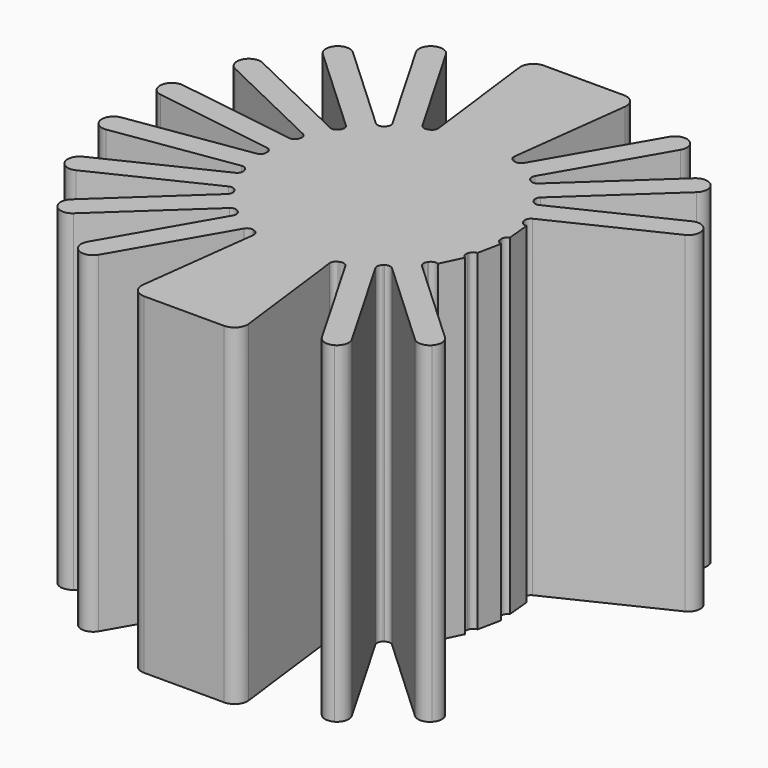
from build123d import *

# Parameters (mm, degrees)
F1_DEPTH = 14
F2_R     = 0.49999
F3_R     = 0.25
F4_R     = 0.55
F6_DEPTH = 14.001


# Not quite as in the source:
# - a fillet or chamfer is up to 0.001 mm smaller than in the source, because OpenCascade refuses the exact size
# - ends of sketch curves that miss each other by under 0.0002 mm in the source are joined


with BuildPart() as f1:
    # F0 (on Top) → F1 (new body)
    with BuildSketch(Plane.XY):
        with BuildLine():
            ThreePointArc((4.9441205719, -0.2411882471), (4.9485299247, -0.1206299488), (4.95, 0))
            ThreePointArc((4.95, 0), (4.9485691313, 0.1190107267), (4.9442773523, 0.2379526499))
            ThreePointArc((4.9442773523, 0.2379526499), (4.894953731, 0.7361575721), (4.7955586509, 1.2268321915))
            ThreePointArc((4.7955586509, 1.2268321915), (4.7305625494, 1.4574902971), (4.6544792073, 1.6847324146))
            ThreePointArc((4.6544792073, 1.6847324146), (4.4604984174, 2.1462650974), (4.2208902988, 2.585843206))
            ThreePointArc((4.2208902988, 2.585843206), (4.0907941216, 2.7870958819), (3.9511101589, 2.9818163109))
            ThreePointArc((3.9511101589, 2.9818163109), (3.6297082448, 3.36566755), (3.2711773205, 3.7150907038))
            ThreePointArc((3.2711773205, 3.7150907038), (3.0875406838, 3.8690557667), (2.8966676337, 4.0139527426))
            ThreePointArc((2.8966676337, 4.0139527426), (2.476402566, 4.2860156709), (2.030805882, 4.5142360893))
            ThreePointArc((2.030805882, 4.5142360893), (1.8088052095, 4.6076809475), (1.5825217056, 4.6902158854))
            ThreePointArc((1.5825217056, 4.6902158854), (0, 4.95), (-1.5825217056, 4.6902158854))
            ThreePointArc((-1.5825217056, 4.6902158854), (-1.8088052095, 4.6076809475), (-2.030805882, 4.5142360893))
            ThreePointArc((-2.030805882, 4.5142360893), (-2.476402566, 4.2860156709), (-2.8966676337, 4.0139527426))
            ThreePointArc((-2.8966676337, 4.0139527426), (-3.0875406838, 3.8690557667), (-3.2711773205, 3.7150907038))
            ThreePointArc((-3.2711773205, 3.7150907038), (-3.6297082448, 3.36566755), (-3.9511101589, 2.9818163109))
            ThreePointArc((-3.9511101589, 2.9818163109), (-4.0907941216, 2.7870958819), (-4.2208902988, 2.585843206))
            ThreePointArc((-4.2208902988, 2.585843206), (-4.4604984174, 2.1462650974), (-4.6544792073, 1.6847324146))
            ThreePointArc((-4.6544792073, 1.6847324146), (-4.7305625494, 1.4574902971), (-4.7955586509, 1.2268321915))
            ThreePointArc((-4.7955586509, 1.2268321915), (-4.894953731, 0.7361575721), (-4.9442773523, 0.2379526499))
            ThreePointArc((-4.9442773523, 0.2379526499), (-4.949999735, -0.0016196967), (-4.9441205719, -0.2411882471))
            ThreePointArc((-4.9441205719, -0.2411882471), (-4.8944709245, -0.7393607841), (-4.7947547569, -1.229970252))
            ThreePointArc((-4.7947547569, -1.229970252), (-4.7296077214, -1.4605857733), (-4.6533756832, -1.6877780515))
            ThreePointArc((-4.6533756832, -1.6877780515), (-4.4590928973, -2.14918369), (-4.21919716, -2.5886048994))
            ThreePointArc((-4.21919716, -2.5886048994), (-4.0889693063, -2.7897723944), (-3.949157944, -2.9844013693))
            ThreePointArc((-3.949157944, -2.9844013693), (-3.6275048978, -3.3680421934), (-3.2687453797, -3.7172306416))
            ThreePointArc((-3.2687453797, -3.7172306416), (-3.0850080241, -3.8710754954), (-2.894040191, -4.0158475286))
            ThreePointArc((-2.894040191, -4.0158475286), (-2.473597169, -4.2876353676), (-2.0278512278, -4.5155641284))
            ThreePointArc((-2.0278512278, -4.5155641284), (-1.8072974267, -4.6082725626), (-1.5825217056, -4.6902158854))
            ThreePointArc((-1.5825217056, -4.6902158854), (0, -4.95), (1.5825217056, -4.6902158854))
            ThreePointArc((1.5825217056, -4.6902158854), (1.8072974267, -4.6082725626), (2.0278512278, -4.5155641284))
            ThreePointArc((2.0278512278, -4.5155641284), (2.473597169, -4.2876353676), (2.894040191, -4.0158475286))
            ThreePointArc((2.894040191, -4.0158475286), (3.0850080241, -3.8710754954), (3.2687453797, -3.7172306416))
            ThreePointArc((3.2687453797, -3.7172306416), (3.6275048978, -3.3680421934), (3.949157944, -2.9844013693))
            ThreePointArc((3.949157944, -2.9844013693), (4.0889693063, -2.7897723944), (4.21919716, -2.5886048994))
            ThreePointArc((4.21919716, -2.5886048994), (4.4590928973, -2.14918369), (4.6533756832, -1.6877780515))
            ThreePointArc((4.6533756832, -1.6877780515), (4.7296077214, -1.4605857733), (4.7947547569, -1.229970252))
            ThreePointArc((4.7947547569, -1.229970252), (4.8944709245, -0.7393607841), (4.9441205719, -0.2411882471))
        make_face()
        with BuildLine():
            ThreePointArc((-3.9511101589, 2.9818163109), (-3.6297082448, 3.36566755), (-3.2711773205, 3.7150907038))
            Line((-3.2711773205, 3.7150907038), (-7.5709054994, 7.7020380367))
            ThreePointArc((-7.5709054994, 7.7020380367), (-7.9193634433, 7.3432746546), (-8.2508383378, 6.9687636438))
            Line((-8.2508383378, 6.9687636438), (-3.9511101589, 2.9818163109))
        make_face()
        with BuildLine():
            ThreePointArc((-2.8966676337, 4.0139527426), (-2.476402566, 4.2860156709), (-2.030805882, 4.5142360893))
            Line((-2.030805882, 4.5142360893), (-4.9643358456, 9.5914216679))
            ThreePointArc((-4.9643358456, 9.5914216679), (-5.403060144, 9.3513069183), (-5.8301975973, 9.0911383213))
            Line((-5.8301975973, 9.0911383213), (-2.8966676337, 4.0139527426))
        make_face()
        with BuildLine():
            ThreePointArc((-1.5825217056, 4.6902158854), (0, 4.95), (1.5825217056, 4.6902158854))
            Line((1.5825217056, 4.6902158854), (2.3103030104, 10.55))
            Line((2.3103030104, 10.55), (-2.3103030104, 10.55))
            Line((-2.3103030104, 10.55), (-1.5825217056, 4.6902158854))
        make_face()
        with BuildLine():
            ThreePointArc((2.030805882, 4.5142360893), (2.476402566, 4.2860156709), (2.8966676337, 4.0139527426))
            Line((2.8966676337, 4.0139527426), (5.8301975973, 9.0911383213))
            ThreePointArc((5.8301975973, 9.0911383213), (5.403060144, 9.3513069183), (4.9643358456, 9.5914216679))
            Line((4.9643358456, 9.5914216679), (2.030805882, 4.5142360893))
        make_face()
        with BuildLine():
            ThreePointArc((3.2711773205, 3.7150907038), (3.6297082448, 3.36566755), (3.9511101589, 2.9818163109))
            Line((3.9511101589, 2.9818163109), (8.2508383378, 6.9687636438))
            ThreePointArc((8.2508383378, 6.9687636438), (7.9193634433, 7.3432746546), (7.5709054994, 7.7020380367))
            Line((7.5709054994, 7.7020380367), (3.2711773205, 3.7150907038))
        make_face()
        with BuildLine():
            ThreePointArc((4.2208902988, 2.585843206), (4.4604984174, 2.1462650974), (4.6544792073, 1.6847324146))
            Line((4.6544792073, 1.6847324146), (9.9383558838, 4.2271837347))
            ThreePointArc((9.9383558838, 4.2271837347), (9.7319965471, 4.6827602124), (9.5047669753, 5.128294526))
            Line((9.5047669753, 5.128294526), (4.2208902988, 2.585843206))
        make_face()
        with BuildLine():
            ThreePointArc((4.7955586509, 1.2268321915), (4.894953731, 0.7361575721), (4.9442773523, 0.2379526499))
            Line((4.9442773523, 0.2379526499), (10.7428068958, 1.11))
            ThreePointArc((10.7428068958, 1.11), (10.6798990496, 1.6061619754), (10.5940881944, 2.0988795416))
            Line((10.5940881944, 2.0988795416), (4.7955586509, 1.2268321915))
        make_face()
        with BuildLine():
            Line((10.742078186, -1.1170301009), (4.9441205719, -0.2411882471))
            ThreePointArc((4.9441205719, -0.2411882471), (4.8944709245, -0.7393607841), (4.7947547569, -1.229970252))
            Line((4.7947547569, -1.229970252), (10.592712371, -2.1058121058))
            ThreePointArc((10.592712371, -2.1058121058), (10.6788456535, -1.6131508017), (10.742078186, -1.1170301009))
        make_face()
        with BuildLine():
            Line((9.93558739, -4.2336867169), (4.6533756832, -1.6877780515))
            ThreePointArc((4.6533756832, -1.6877780515), (4.4590928973, -2.14918369), (4.21919716, -2.5886048994))
            Line((4.21919716, -2.5886048994), (9.5014088667, -5.1345135648))
            ThreePointArc((9.5014088667, -5.1345135648), (9.7289299578, -4.6891280508), (9.93558739, -4.2336867169))
        make_face()
        with BuildLine():
            Line((8.2462760527, -6.9741616889), (3.949157944, -2.9844013693))
            ThreePointArc((3.949157944, -2.9844013693), (3.6275048978, -3.3680421934), (3.2687453797, -3.7172306416))
            Line((3.2687453797, -3.7172306416), (7.5658634884, -7.7069909611))
            ThreePointArc((7.5658634884, -7.7069909611), (7.9145561406, -7.3484556947), (8.2462760527, -6.9741616889))
        make_face()
        with BuildLine():
            Line((5.8242469, -9.0949517892), (2.894040191, -4.0158475286))
            ThreePointArc((2.894040191, -4.0158475286), (2.473597169, -4.2876353676), (2.0278512278, -4.5155641284))
            Line((2.0278512278, -4.5155641284), (4.9580579369, -9.594668389))
            ThreePointArc((4.9580579369, -9.594668389), (5.3969392779, -9.354840802), (5.8242469, -9.0949517892))
        make_face()
        with BuildLine():
            Line((2.3103030104, -10.55), (1.5825217056, -4.6902158854))
            ThreePointArc((1.5825217056, -4.6902158854), (0, -4.95), (-1.5825217056, -4.6902158854))
            Line((-1.5825217056, -4.6902158854), (-2.3103030104, -10.55))
            Line((-2.3103030104, -10.55), (2.3103030104, -10.55))
        make_face()
        with BuildLine():
            Line((-7.5658634884, -7.7069909611), (-3.2687453797, -3.7172306416))
            ThreePointArc((-3.2687453797, -3.7172306416), (-3.6275048978, -3.3680421934), (-3.949157944, -2.9844013693))
            Line((-3.949157944, -2.9844013693), (-8.2462760527, -6.9741616889))
            ThreePointArc((-8.2462760527, -6.9741616889), (-7.9145561406, -7.3484556947), (-7.5658634884, -7.7069909611))
        make_face()
        with BuildLine():
            Line((-4.9580579369, -9.594668389), (-2.0278512278, -4.5155641284))
            ThreePointArc((-2.0278512278, -4.5155641284), (-2.473597169, -4.2876353676), (-2.894040191, -4.0158475286))
            Line((-2.894040191, -4.0158475286), (-5.8242469, -9.0949517892))
            ThreePointArc((-5.8242469, -9.0949517892), (-5.3969392779, -9.354840802), (-4.9580579369, -9.594668389))
        make_face()
        with BuildLine():
            Line((-9.5014088667, -5.1345135648), (-4.21919716, -2.5886048994))
            ThreePointArc((-4.21919716, -2.5886048994), (-4.4590928973, -2.14918369), (-4.6533756832, -1.6877780515))
            Line((-4.6533756832, -1.6877780515), (-9.93558739, -4.2336867169))
            ThreePointArc((-9.93558739, -4.2336867169), (-9.7289299578, -4.6891280508), (-9.5014088667, -5.1345135648))
        make_face()
        with BuildLine():
            Line((-10.592712371, -2.1058121058), (-4.7947547569, -1.229970252))
            ThreePointArc((-4.7947547569, -1.229970252), (-4.8944709245, -0.7393607841), (-4.9441205719, -0.2411882471))
            Line((-4.9441205719, -0.2411882471), (-10.742078186, -1.1170301009))
            ThreePointArc((-10.742078186, -1.1170301009), (-10.6788456535, -1.6131508017), (-10.592712371, -2.1058121058))
        make_face()
        with BuildLine():
            ThreePointArc((-4.9442773523, 0.2379526499), (-4.894953731, 0.7361575721), (-4.7955586509, 1.2268321915))
            Line((-4.7955586509, 1.2268321915), (-10.5940881944, 2.0988795416))
            ThreePointArc((-10.5940881944, 2.0988795416), (-10.6798990496, 1.6061619754), (-10.7428068958, 1.11))
            Line((-10.7428068958, 1.11), (-4.9442773523, 0.2379526499))
        make_face()
        with BuildLine():
            ThreePointArc((-4.6544792073, 1.6847324146), (-4.4604984174, 2.1462650974), (-4.2208902988, 2.585843206))
            Line((-4.2208902988, 2.585843206), (-9.5047669753, 5.128294526))
            ThreePointArc((-9.5047669753, 5.128294526), (-9.7319965471, 4.6827602124), (-9.9383558838, 4.2271837347))
            Line((-9.9383558838, 4.2271837347), (-4.6544792073, 1.6847324146))
        make_face()
    extrude(amount=F1_DEPTH)

    # F2 (radius 0.5 in the source; OpenCascade refuses exactly that, so slightly less here)
    f2_edges = [f1.edges().sort_by_distance(p)[0] for p in [
        (-4.958058, -9.594668, 7),
        (-5.824247, -9.094952, 7),
        (-7.565863, -7.706991, 7),
        (-8.246276, -6.974162, 7),
        (-9.501409, -5.134514, 7),
        (-9.935587, -4.233687, 7),
        (-10.592712, -2.105812, 7),
        (-10.742078, -1.11703, 7),
        (-10.742807, 1.11, 7),
        (-10.594088, 2.09888, 7),
        (-9.938356, 4.227184, 7),
        (-9.504767, 5.128295, 7),
        (-8.250838, 6.968764, 7),
        (-7.570905, 7.702038, 7),
        (-4.964336, 9.591422, 7),
        (-5.830198, 9.091138, 7),
        (4.964336, 9.591422, 7),
        (5.830198, 9.091138, 7),
        (7.570905, 7.702038, 7),
        (8.250838, 6.968764, 7),
        (9.938356, 4.227184, 7),
        (9.504767, 5.128295, 7),
        (10.742807, 1.11, 7),
        (10.594088, 2.09888, 7),
        (10.592712, -2.105812, 7),
        (10.742078, -1.11703, 7),
        (9.501409, -5.134514, 7),
        (9.935587, -4.233687, 7),
        (7.565863, -7.706991, 7),
        (8.246276, -6.974162, 7),
        (4.958058, -9.594668, 7),
        (5.824247, -9.094952, 7),
    ]]
    fillet(f2_edges, radius=F2_R)

    # F3
    f3_edges = [f1.edges().sort_by_distance(p)[0] for p in [
        (-2.027851, -4.515564, 7),
        (-1.582522, -4.690216, 7),
        (-2.89404, -4.015848, 7),
        (-3.268745, -3.717231, 7),
        (-4.219197, -2.588605, 7),
        (-3.949158, -2.984401, 7),
        (-4.794755, -1.22997, 7),
        (-4.653376, -1.687778, 7),
        (-4.944277, 0.237953, 7),
        (-4.944121, -0.241188, 7),
        (-4.654479, 1.684732, 7),
        (-4.795559, 1.226832, 7),
        (-4.22089, 2.585843, 7),
        (-3.95111, 2.981816, 7),
        (-2.896668, 4.013953, 7),
        (-3.271177, 3.715091, 7),
        (-1.582522, 4.690216, 7),
        (-2.030806, 4.514236, 7),
        (2.030806, 4.514236, 7),
        (1.582522, 4.690216, 7),
        (2.896668, 4.013953, 7),
        (3.271177, 3.715091, 7),
        (3.95111, 2.981816, 7),
        (4.22089, 2.585843, 7),
        (4.654479, 1.684732, 7),
        (4.944277, 0.237953, 7),
        (4.944121, -0.241188, 7),
        (4.795559, 1.226832, 7),
        (4.794755, -1.22997, 7),
        (4.653376, -1.687778, 7),
        (3.949158, -2.984401, 7),
        (4.219197, -2.588605, 7),
        (3.268745, -3.717231, 7),
        (2.027851, -4.515564, 7),
        (1.582522, -4.690216, 7),
        (2.89404, -4.015848, 7),
    ]]
    fillet(f3_edges, radius=F3_R)

    # F4
    f4_edges = [f1.edges().sort_by_distance(p)[0] for p in [
        (2.310303, -10.55, 7),
        (-2.310303, -10.55, 7),
        (-2.310303, 10.55, 7),
        (2.310303, 10.55, 7),
    ]]
    fillet(f4_edges, radius=F4_R)

    # F5 (on face) → F6 (cut, through all)
    with BuildSketch(Plane.XY.offset(14)):
        with BuildLine():
            Line((4.8524102064, -1.7837082689), (4.4182316832, -2.6845351168))
            Line((4.4182316832, -2.6845351168), (9.0614362804, -4.922456555))
            ThreePointArc((9.0614362804, -4.922456555), (9.4435027689, -4.9440384549), (9.7289254052, -4.6891374964))
            ThreePointArc((9.7289254052, -4.6891374964), (9.7505160393, -4.3070520959), (9.4956148037, -4.021629707))
            Line((9.4956148037, -4.021629707), (4.8524102064, -1.7837082689))
        make_face()
        with BuildLine():
            Line((5.1625884777, -0.2741900985), (4.9598829093, -1.260680021))
            ThreePointArc((4.9598829093, -1.260680021), (4.9866141474, -1.2603981029), (5.0132226627, -1.2629721034))
            Line((5.0132226627, -1.2629721034), (10.1097816313, -2.0328603903))
            ThreePointArc((10.1097816313, -2.0328603903), (10.4812353544, -1.9408673925), (10.6788440873, -1.6131611695))
            ThreePointArc((10.6788440873, -1.6131611695), (10.5868538612, -1.2416868002), (10.2591474463, -1.0440783854))
            Line((10.2591474463, -1.0440783854), (5.1625884777, -0.2741900985))
        make_face()
        with BuildLine():
            Line((5.014048107, 1.2596910654), (5.1111211874, 0.2572796071))
            ThreePointArc((5.1111211874, 0.2572796071), (5.1365817348, 0.2654281712), (5.1627668085, 0.2708115238))
            Line((5.1627668085, 0.2708115238), (10.2598285183, 1.0373643411))
            ThreePointArc((10.2598285183, 1.0373643411), (10.5876641825, 1.234758255), (10.6799006089, 1.6061516066))
            ThreePointArc((10.6799006089, 1.6061516066), (10.482503258, 1.9340078168), (10.1111098168, 2.0262438827))
            Line((10.1111098168, 2.0262438827), (5.014048107, 1.2596910654))
        make_face()
    extrude(amount=-F6_DEPTH, mode=Mode.SUBTRACT)


solid = f1.part
